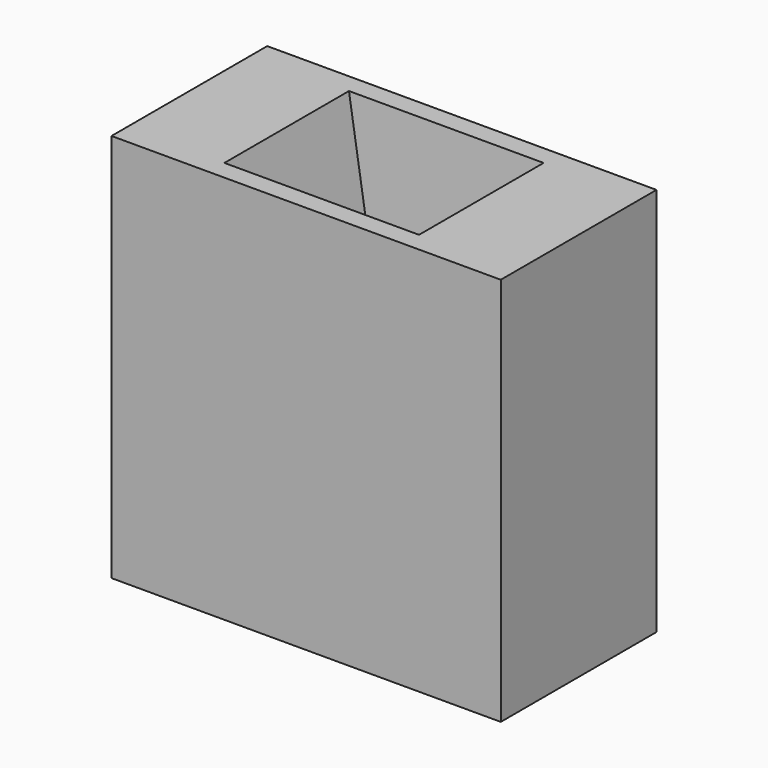
from build123d import *

# Parameters (mm, degrees)
F0_W     = 2
F0_H     = 1
F1_DEPTH = 2
F2_W     = 1
F2_H     = 0.8
F3_W     = 0.1
F3_H     = 0.5


with BuildPart() as f1:
    # F0 (on Top) → F1 (new body)
    with BuildSketch(Plane.XY):
        with Locations((55.8135678768, -38.8856279552)):
            Rectangle(F0_W, F0_H)
    extrude(amount=F1_DEPTH)

    # F2 (on face) → F4 section 0
    with BuildSketch(Plane.XY.offset(2)):
        with Locations((55.8135678768, -38.8856279552)):
            Rectangle(F2_W, F2_H)
    # F3 (on face) → F4 section 1
    with BuildSketch(Plane(origin=(0, 0, 0), x_dir=(1, 0, 0), z_dir=(0, 0, -1))):
        with Locations((55.8135678768, 38.8856279552)):
            Rectangle(F3_W, F3_H)
    loft(mode=Mode.SUBTRACT)


solid = f1.part
